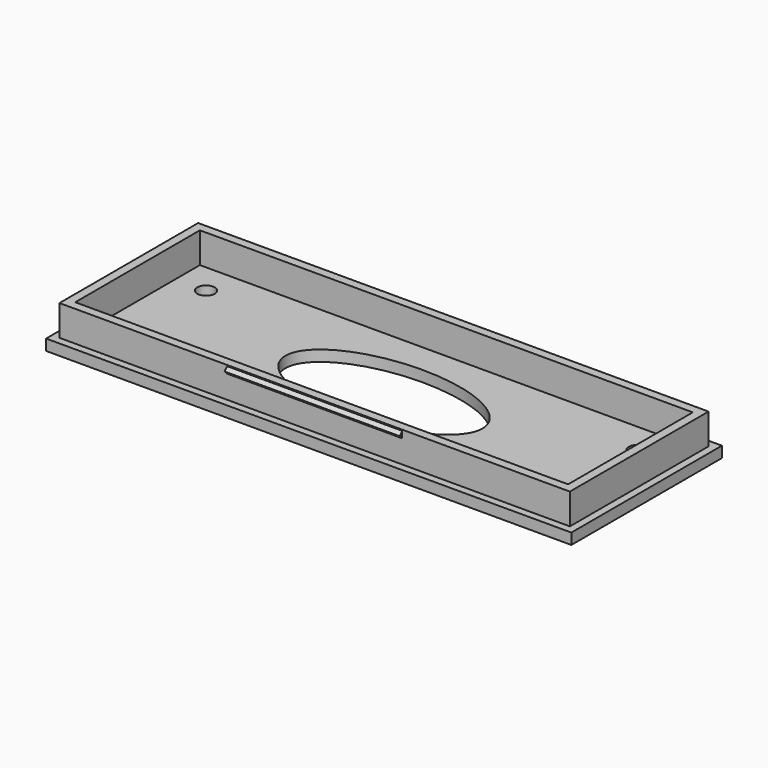
from build123d import *

# Parameters (mm, degrees)
F0_W        = 120
F0_H        = 43
F0_W_2      = 116.6
F0_H_2      = 39.6
F0_W_3      = 112.6
F0_H_3      = 35.6
F0_R        = 2
F1_DEPTH    = 2.5
F2_DEPTH    = 7
F3_W        = 40
F3_H        = 1.5
F4_DEPTH    = 0.8
F5_T4_DEPTH = 44.1146927807
F5_T9_DEPTH = 44.1146927807


# Not quite as in the source:
# - a fillet or chamfer that OpenCascade refuses, or shapes differently, is made with other operations: its cross-section is extruded or revolved along the edge and cut away or added


with BuildPart() as f1:
    # F0 (on Top) → F1 (new body)
    with BuildSketch(Plane.XY):
        Rectangle(F0_W, F0_H)
        Rectangle(F0_W_2, F0_H_2, mode=Mode.SUBTRACT)
        Rectangle(F0_W_2, F0_H_2)
        Rectangle(F0_W_3, F0_H_3, mode=Mode.SUBTRACT)
        Rectangle(F0_W_3, F0_H_3)
        with Locations((-49.3, -10.8)):
            Circle(F0_R, mode=Mode.SUBTRACT)
        with Locations((49.3, -10.8)):
            Circle(F0_R, mode=Mode.SUBTRACT)
        with Locations((-49.3, 10.8)):
            Circle(F0_R, mode=Mode.SUBTRACT)
        with BuildLine():
            add(Edge.make_bspline(
                [(22.5, 0), (22.5, 19.0525588833), (-11.25, 9.5262794416), (-45, 0), (-11.25, -9.5262794416), (22.5, -19.0525588833), (22.5, 0)],
                knots=[0, 0, 0, 2.0943951024, 2.0943951024, 4.1887902048, 4.1887902048, 6.2831853072, 6.2831853072, 6.2831853072], degree=2, weights=[1, 0.5, 1, 0.5, 1, 0.5, 1]))
        make_face(mode=Mode.SUBTRACT)
        with Locations((49.3, 10.8)):
            Circle(F0_R, mode=Mode.SUBTRACT)
    extrude(amount=-F1_DEPTH)

    # F0 (on Top) → F2 (join)
    with BuildSketch(Plane.XY):
        Rectangle(F0_W_2, F0_H_2)
        Rectangle(F0_W_3, F0_H_3, mode=Mode.SUBTRACT)
    extrude(amount=F2_DEPTH)

    # F3 (on face) → F4 (join)
    with BuildSketch(Plane(origin=(0, 19.8, 0), x_dir=(-1, 0, 0), z_dir=(0, 1, 0))):
        with Locations((0, 6)):
            Rectangle(F3_W, F3_H)
    extrude(amount=F4_DEPTH)

    # F5: chamfer of 0.8 on 2 edges, made by hand


with BuildPart() as f5_tool2:
    # F5_s3 → F5_t4 (new body)
    with BuildSketch(Plane.YZ.offset(22.0573463904)):
        Polygon((19.8, 5.25), (20.6, 6.05), (20.6, 5.25), align=None)
    extrude(amount=-F5_T4_DEPTH)

    split(bisect_by=Plane.XZ.offset(-19.8), keep=Keep.BOTTOM)


with BuildPart() as f1_1:
    add(f1.part)

    # F5_t1: cut F5_tool2
    add(f5_tool2.part, mode=Mode.SUBTRACT)


with BuildPart() as f5_tool7:
    # F5_s8 → F5_t9 (new body)
    with BuildSketch(Plane.YZ.offset(-22.0573463904)):
        Polygon((19.8, 6.75), (20.6, 5.95), (20.6, 6.75), align=None)
    extrude(amount=F5_T9_DEPTH)

    split(bisect_by=Plane.XZ.offset(-19.8), keep=Keep.BOTTOM)


with BuildPart() as f1_2:
    add(f1_1.part)

    # F5_t6: cut F5_tool7
    add(f5_tool7.part, mode=Mode.SUBTRACT)

    # F6: F1 across plane


with BuildPart() as f1_3:
    add(f1_2.part)
    add(f1_2.part.mirror(Plane.XZ))


solid = f1_3.part
